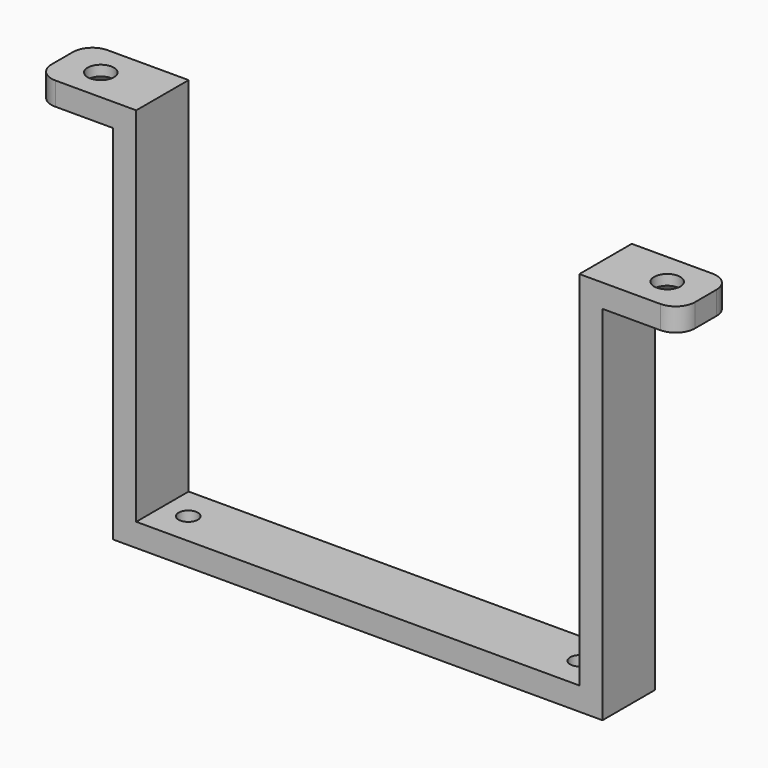
from build123d import *

# Parameters (mm, degrees)
F0_W            = 63.5
F0_H            = 8.5
F0_R            = 1.25
F1_DEPTH        = 3
F2_W            = 3
F2_H            = 8.5
F3_DEPTH        = 47
F4_W            = 8.5
F4_H            = 3
F5_DEPTH        = 10
F6_W            = 8.5
F6_H            = 3
F7_DEPTH        = 10
F9_D            = 3.4
F9_DEPTH        = 5
F9_CSINK_D      = 6.72
F9_CSINK_ANGLE  = 90
F9_TIP          = 1.0214630523
F11_D           = 3.4
F11_DEPTH       = 5
F11_CSINK_D     = 6.72
F11_CSINK_ANGLE = 90
F11_TIP         = 1.0214630523
F12_R           = 2.5


with BuildPart() as f1:
    # F0 (on Top) → F1 (new body)
    with BuildSketch(Plane.XY):
        Rectangle(F0_W, F0_H)
        with Locations((-25.4, 0)):
            Circle(F0_R, mode=Mode.SUBTRACT)
        with Locations((25.4, 0)):
            Circle(F0_R, mode=Mode.SUBTRACT)
    extrude(amount=F1_DEPTH)

    # F2 (on face) → F3 (join)
    with BuildSketch(Plane.XY.offset(3)):
        with Locations((-30.25, 0)):
            Rectangle(F2_W, F2_H)
        with Locations((30.25, 0)):
            Rectangle(F2_W, F2_H)
    extrude(amount=F3_DEPTH)

    # F4 (on face) → F5 (join)
    with BuildSketch(Plane(origin=(-31.75, 0, 0), x_dir=(0, -1, 0), z_dir=(-1, 0, 0))):
        with Locations((0, 48.5)):
            Rectangle(F4_W, F4_H)
    extrude(amount=F5_DEPTH)

    # F6 (on face) → F7 (join)
    with BuildSketch(Plane.YZ.offset(31.75)):
        with Locations((0, 48.5)):
            Rectangle(F6_W, F6_H)
    extrude(amount=F7_DEPTH)

    # F9
    with Locations(Plane(origin=(0, 0, 47), x_dir=(1, 0, 0), z_dir=(0, 0, -1))):
        with Locations((-36.75, 0)):
            CounterSinkHole(F9_D / 2, F9_CSINK_D / 2, depth=F9_DEPTH, counter_sink_angle=F9_CSINK_ANGLE)
            with Locations((0, 0, -(F9_DEPTH + F9_TIP / 2))):  # 118° drill point
                Cone(0, F9_D / 2, F9_TIP, mode=Mode.SUBTRACT)

    # F11
    with Locations(Plane(origin=(0, 0, 47), x_dir=(1, 0, 0), z_dir=(0, 0, -1))):
        with Locations((36.75, 0)):
            CounterSinkHole(F11_D / 2, F11_CSINK_D / 2, depth=F11_DEPTH, counter_sink_angle=F11_CSINK_ANGLE)
            with Locations((0, 0, -(F11_DEPTH + F11_TIP / 2))):  # 118° drill point
                Cone(0, F11_D / 2, F11_TIP, mode=Mode.SUBTRACT)

    # F12
    f12_edges = [f1.edges().sort_by_distance(p)[0] for p in [
        (41.75, 4.25, 48.5),
        (41.75, -4.25, 48.5),
        (-41.75, 4.25, 48.5),
        (-41.75, -4.25, 48.5),
    ]]
    fillet(f12_edges, radius=F12_R)


solid = f1.part
